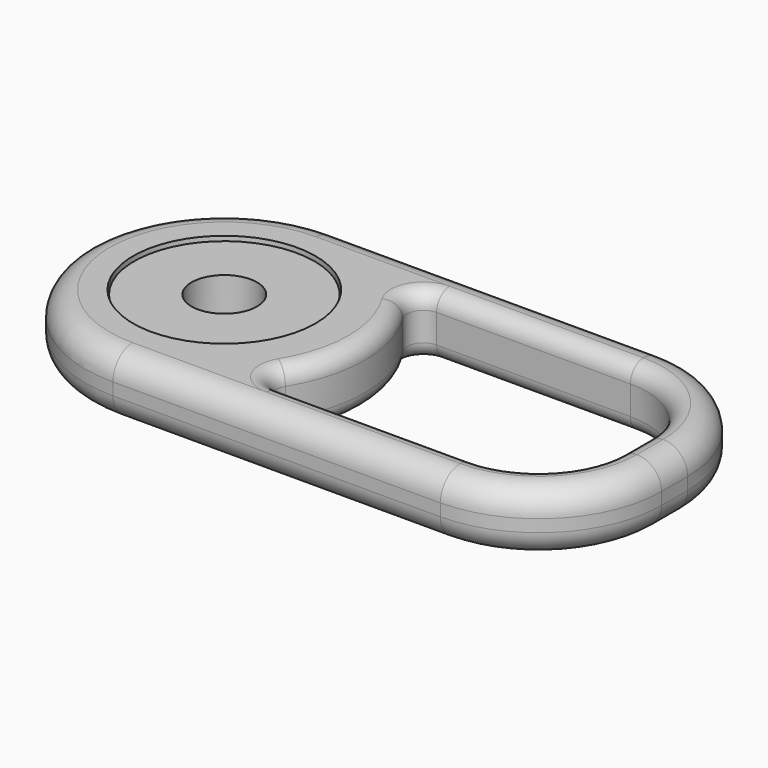
from build123d import *

# Parameters (mm, degrees)
F0_R     = 11
F0_R_2   = 4
F1_DEPTH = 7
F2_R     = 11.15
F3_DEPTH = 7.5
F4_R     = 3
F6_DEPTH = 25
F7_R     = 1.99999


# Not quite as in the source:
# - a fillet or chamfer is up to 0.001 mm smaller than in the source, because OpenCascade refuses the exact size


with BuildPart() as f1:
    # F0 (on Top) → F1 (new body)
    with BuildSketch(Plane.XY):
        Circle(F0_R)
        Circle(F0_R_2, mode=Mode.SUBTRACT)
    extrude(amount=F1_DEPTH)


with BuildPart() as f3:
    # F2 (on Top) → F3 (new body)
    with BuildSketch(Plane.XY):
        with BuildLine():
            Line((40, 17), (0, 17))
            ThreePointArc((0, 17), (-17, 0), (0, -17))
            Line((0, -17), (40, -17))
            ThreePointArc((40, -17), (50.6066017178, -12.6066017178), (55, -2))
            Line((55, -2), (55, 2))
            ThreePointArc((55, 2), (50.6066017178, 12.6066017178), (40, 17))
        make_face()
        Circle(F2_R, mode=Mode.SUBTRACT)
    extrude(amount=F3_DEPTH)

    # F4
    f4_edges = [f3.edges().sort_by_distance(p)[0] for p in [
        (20, -17, 7.5),
        (50.606602, -12.606602, 7.5),
        (20, -17, 0),
        (20, 17, 0),
        (20, 17, 7.5),
        (-17, 0, 0),
        (-17, 0, 7.5),
        (50.606602, -12.606602, 0),
        (55, 0, 0),
        (55, 0, 7.5),
        (50.606602, 12.606602, 0),
        (50.606602, 12.606602, 7.5),
    ]]
    fillet(f4_edges, radius=F4_R)

    # F5 (on face) → F6 (cut)
    with BuildSketch(Plane(origin=(0, 0, 0), x_dir=(1, 0, 0), z_dir=(0, 0, -1))):
        with BuildLine():
            ThreePointArc((50, 2), (47.0710678119, 9.0710678119), (40, 12))
            Line((40, 12), (12.2524487348, 12))
            ThreePointArc((12.2524487348, 12), (17.15, 0), (12.2524487348, -12))
            Line((12.2524487348, -12), (40, -12))
            ThreePointArc((40, -12), (47.0710678119, -9.0710678119), (50, -2))
            Line((50, -2), (50, 2))
        make_face()
    extrude(amount=-F6_DEPTH, mode=Mode.SUBTRACT)

    # F7 (radius 2 in the source; OpenCascade refuses exactly that, so slightly less here)
    f7_edges = [f3.edges().sort_by_distance(p)[0] for p in [
        (26.126224, -12, 0),
        (12.252449, -12, 3.75),
        (47.071068, -9.071068, 7.5),
        (47.071068, 9.071068, 7.5),
        (26.126224, 12, 7.5),
        (47.071068, 9.071068, 0),
        (26.126224, 12, 0),
        (47.071068, -9.071068, 0),
        (50, 0, 7.5),
        (50, 0, 0),
        (12.252449, 12, 3.75),
        (17.15, 0, 0),
        (17.15, 0, 7.5),
        (26.126224, -12, 7.5),
    ]]
    fillet(f7_edges, radius=F7_R)


solid = Compound([f1.part, f3.part])
